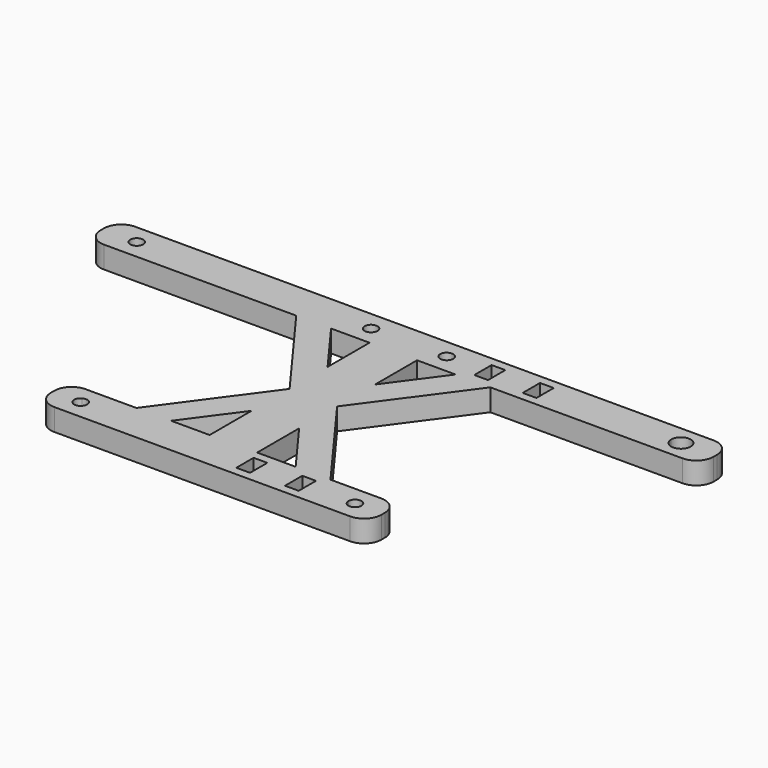
from build123d import *

# Parameters (mm, degrees)
F1_DEPTH = 5.08
F2_R     = 4


# Not quite as in the source:
# - a feature names something its author has since deleted; it is built from what else it names


with BuildPart() as f1:
    # F0 (on Top) → F1 (new body)
    with BuildSketch(Plane.XY):
        with BuildLine():
            Line((0.6656670719, 55.2782733088), (-50.5843329281, 55.2782733088))
            ThreePointArc((-50.5843329281, 55.2782733088), (-50.7887088575, 54.5223908657), (-51.3461439517, 53.9724873251))
            Line((-51.3461439517, 53.9724873251), (-49.5403858838, 50.7782733088))
            Line((-49.5403858838, 50.7782733088), (-11.5572661318, 50.7782733088))
            Line((-11.5572661318, 50.7782733088), (-3.4960969558, 50.7782733088))
            Line((-3.4960969558, 50.7782733088), (5.4156670719, 50.7782733088))
            Line((5.4156670719, 50.7782733088), (10.9156670719, 50.7782733088))
            Line((10.9156670719, 50.7782733088), (10.9156670719, 55.2782733088))
            Line((10.9156670719, 55.2782733088), (3.6656670719, 55.2782733088))
            ThreePointArc((3.6656670719, 55.2782733088), (2.1656670719, 53.7782733088), (0.6656670719, 55.2782733088))
        make_face()
        with BuildLine():
            Line((-11.5572661318, 4.5), (-23.3782799724, 4.5))
            Line((-23.3782799724, 4.5), (-21.5725219045, 1.3057859837))
            ThreePointArc((-21.5725219045, 1.3057859837), (-20.0784504851, 1.2956240706), (-19.3343329281, 0))
            Line((-19.3343329281, 0), (10.9156670719, 0))
            Line((10.9156670719, 0), (10.9156670719, 4.5))
            Line((10.9156670719, 4.5), (5.4156670719, 4.5))
            Line((5.4156670719, 4.5), (-3.4960969558, 4.5))
            Line((-3.4960969558, 4.5), (-11.5572661318, 4.5))
        make_face()
        with BuildLine():
            ThreePointArc((-51.3461439517, 53.9724873251), (-53.3799569987, 56.0341557518), (-50.5843329281, 55.2782733088))
            Line((-50.5843329281, 55.2782733088), (0.6656670719, 55.2782733088))
            ThreePointArc((0.6656670719, 55.2782733088), (2.1656670719, 56.7782733088), (3.6656670719, 55.2782733088))
            Line((3.6656670719, 55.2782733088), (10.9156670719, 55.2782733088))
            Line((10.9156670719, 55.2782733088), (18.1656670719, 55.2782733088))
            ThreePointArc((18.1656670719, 55.2782733088), (19.6656670719, 56.7782733088), (21.1656670719, 55.2782733088))
            Line((21.1656670719, 55.2782733088), (28.1048402488, 55.2782733088))
            Line((28.1048402488, 55.2782733088), (28.1048402488, 57.7362733088))
            Line((28.1048402488, 57.7362733088), (31.2798402488, 57.7362733088))
            Line((31.2798402488, 57.7362733088), (31.2798402488, 55.2782733088))
            Line((31.2798402488, 55.2782733088), (39.3168402488, 55.2782733088))
            Line((39.3168402488, 55.2782733088), (39.3168402488, 57.7362733088))
            Line((39.3168402488, 57.7362733088), (42.4918402488, 57.7362733088))
            Line((42.4918402488, 57.7362733088), (42.4918402488, 55.2782733088))
            Line((42.4918402488, 55.2782733088), (71.6656670719, 55.2782733088))
            ThreePointArc((71.6656670719, 55.2782733088), (73.9156670719, 57.5282733088), (76.1656670719, 55.2782733088))
            ThreePointArc((76.1656670719, 55.2782733088), (75.0494907365, 53.3348372029), (72.8083836073, 53.3195943333))
            Line((72.8083836073, 53.3195943333), (71.3717200276, 50.7782733088))
            Line((71.3717200276, 50.7782733088), (81.8841302488, 50.7782733088))
            Line((81.8841302488, 50.7782733088), (81.8841302488, 59.7782733088))
            Line((81.8841302488, 59.7782733088), (-60.052796105, 59.7782733088))
            Line((-60.052796105, 59.7782733088), (-60.052796105, 50.7782733088))
            Line((-60.052796105, 50.7782733088), (-49.5403858838, 50.7782733088))
            Line((-49.5403858838, 50.7782733088), (-51.3461439517, 53.9724873251))
        make_face()
        with BuildLine():
            Line((-21.5725219045, 1.3057859837), (-23.3782799724, 4.5))
            Line((-23.3782799724, 4.5), (-27.3365851734, 4.5))
            Line((-27.3365851734, 4.5), (-27.3365851734, -4.5))
            Line((-27.3365851734, -4.5), (49.1679193172, -4.5))
            Line((49.1679193172, -4.5), (49.1679193172, 4.5))
            Line((49.1679193172, 4.5), (45.2096141162, 4.5))
            Line((45.2096141162, 4.5), (43.4038560483, 1.3057859837))
            ThreePointArc((43.4038560483, 1.3057859837), (43.9612911425, 0.7558824431), (44.1656670719, 0))
            ThreePointArc((44.1656670719, 0), (42.6656670719, -1.5), (41.1656670719, 0))
            Line((41.1656670719, 0), (31.6349193172, 0))
            Line((31.6349193172, 0), (31.6349193172, -2.5))
            Line((31.6349193172, -2.5), (28.4599193172, -2.5))
            Line((28.4599193172, -2.5), (28.4599193172, 0))
            Line((28.4599193172, 0), (20.3669193172, 0))
            Line((20.3669193172, 0), (20.3669193172, -2.5))
            Line((20.3669193172, -2.5), (17.1919193172, -2.5))
            Line((17.1919193172, -2.5), (17.1919193172, 0))
            Line((17.1919193172, 0), (10.9156670719, 0))
            Line((10.9156670719, 0), (-19.3343329281, 0))
            ThreePointArc((-19.3343329281, 0), (-21.5902153712, -1.2956240706), (-21.5725219045, 1.3057859837))
        make_face()
        with BuildLine():
            Line((10.9156670719, 4.5), (10.9156670719, 0))
            Line((10.9156670719, 0), (17.1919193172, 0))
            Line((17.1919193172, 0), (17.1919193172, 2.5))
            Line((17.1919193172, 2.5), (20.3669193172, 2.5))
            Line((20.3669193172, 2.5), (20.3669193172, 0))
            Line((20.3669193172, 0), (28.4599193172, 0))
            Line((28.4599193172, 0), (28.4599193172, 2.5))
            Line((28.4599193172, 2.5), (31.6349193172, 2.5))
            Line((31.6349193172, 2.5), (31.6349193172, 0))
            Line((31.6349193172, 0), (41.1656670719, 0))
            ThreePointArc((41.1656670719, 0), (41.9097846288, 1.2956240706), (43.4038560483, 1.3057859837))
            Line((43.4038560483, 1.3057859837), (45.2096141162, 4.5))
            Line((45.2096141162, 4.5), (33.3886002756, 4.5))
            Line((33.3886002756, 4.5), (25.3274310996, 4.5))
            Line((25.3274310996, 4.5), (16.4156670719, 4.5))
            Line((16.4156670719, 4.5), (10.9156670719, 4.5))
        make_face()
        with BuildLine():
            Line((18.1656670719, 55.2782733088), (10.9156670719, 55.2782733088))
            Line((10.9156670719, 55.2782733088), (10.9156670719, 50.7782733088))
            Line((10.9156670719, 50.7782733088), (16.4156670719, 50.7782733088))
            Line((16.4156670719, 50.7782733088), (25.3274310996, 50.7782733088))
            Line((25.3274310996, 50.7782733088), (33.3886002756, 50.7782733088))
            Line((33.3886002756, 50.7782733088), (71.3717200276, 50.7782733088))
            Line((71.3717200276, 50.7782733088), (72.8083836073, 53.3195943333))
            ThreePointArc((72.8083836073, 53.3195943333), (71.972230966, 54.1444496442), (71.6656670719, 55.2782733088))
            Line((71.6656670719, 55.2782733088), (42.4918402488, 55.2782733088))
            Line((42.4918402488, 55.2782733088), (42.4918402488, 52.7362733088))
            Line((42.4918402488, 52.7362733088), (39.3168402488, 52.7362733088))
            Line((39.3168402488, 52.7362733088), (39.3168402488, 55.2782733088))
            Line((39.3168402488, 55.2782733088), (31.2798402488, 55.2782733088))
            Line((31.2798402488, 55.2782733088), (31.2798402488, 52.7362733088))
            Line((31.2798402488, 52.7362733088), (28.1048402488, 52.7362733088))
            Line((28.1048402488, 52.7362733088), (28.1048402488, 55.2782733088))
            Line((28.1048402488, 55.2782733088), (21.1656670719, 55.2782733088))
            ThreePointArc((21.1656670719, 55.2782733088), (19.6656670719, 53.7782733088), (18.1656670719, 55.2782733088))
        make_face()
        Polygon((5.4156670719, 38.6288985841), (5.4156670719, 27.6391366544), (10.9156670719, 27.6391366544), (10.9156670719, 50.7782733088), (5.4156670719, 50.7782733088), align=None)
        Polygon((10.9156670719, 27.6391366544), (5.4156670719, 27.6391366544), (5.4156670719, 16.6493747247), (5.4156670719, 4.5), (10.9156670719, 4.5), align=None)
        Polygon((16.4156670719, 50.7782733088), (10.9156670719, 50.7782733088), (10.9156670719, 27.6391366544), (16.4156670719, 27.6391366544), (16.4156670719, 38.6288985841), align=None)
        Polygon((16.4156670719, 27.6391366544), (10.9156670719, 27.6391366544), (10.9156670719, 4.5), (16.4156670719, 4.5), (16.4156670719, 16.6493747247), align=None)
        Polygon((-3.4960969558, 50.7782733088), (-11.5572661318, 50.7782733088), (5.4156670719, 27.6391366544), (5.4156670719, 38.6288985841), align=None)
        Polygon((5.4156670719, 27.6391366544), (-11.5572661318, 4.5), (-3.4960969558, 4.5), (5.4156670719, 16.6493747247), align=None)
        Polygon((33.3886002756, 4.5), (16.4156670719, 27.6391366544), (16.4156670719, 16.6493747247), (25.3274310996, 4.5), align=None)
        Polygon((16.4156670719, 38.6288985841), (16.4156670719, 27.6391366544), (33.3886002756, 50.7782733088), (25.3274310996, 50.7782733088), align=None)
    extrude(amount=F1_DEPTH)

    # F2
    f2_edges = [f1.edges().sort_by_distance(p)[0] for p in [
        (-60.052796, 59.778273, 2.54),
        (-60.052796, 50.778273, 2.54),
        (81.88413, 59.778273, 2.54),
        (81.88413, 50.778273, 2.54),
        (49.167919, 4.5, 2.54),
        (49.167919, -4.5, 2.54),
        (-27.336585, 4.5, 2.54),
        (-27.336585, -4.5, 2.54),
    ]]
    fillet(f2_edges, radius=F2_R)


solid = f1.part
